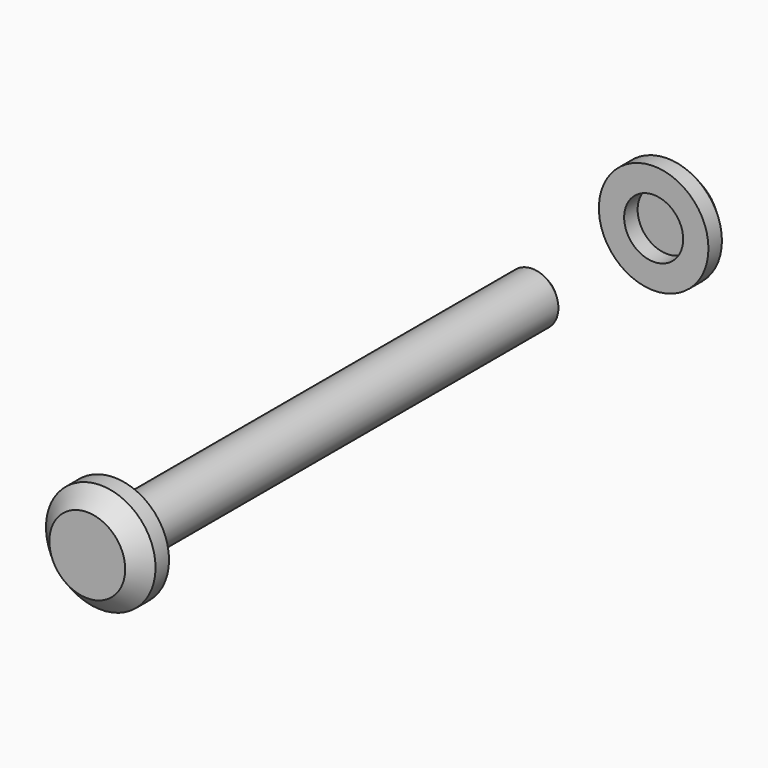
from build123d import *

# Parameters (mm, degrees)
F0_R     = 1.55
F1_DEPTH = 31.5
F0_R_2   = 3.25
F0_R_3   = 1.75
F2_DEPTH = 2
F3_SIZE  = 1
F4_SIZE  = 0.5
F5_START = -40
F5_DEPTH = 2
F6_START = -41
F6_DEPTH = 1
F7_SIZE  = 1


with BuildPart() as f1:
    # F0 (on Front) → F1 (new body)
    with BuildSketch(Plane.XZ):
        Circle(F0_R)
    extrude(amount=-F1_DEPTH)

    # F0 (on Front) → F2 (join)
    with BuildSketch(Plane.XZ):
        Circle(F0_R_2)
        Circle(F0_R_3, mode=Mode.SUBTRACT)
        Circle(F0_R_3)
        Circle(F0_R, mode=Mode.SUBTRACT)
        Circle(F0_R)
    extrude(amount=F2_DEPTH)

    # F3
    f3_edges = [f1.edges().sort_by_distance(p)[0] for p in [
        (-3.25, -2, 0),
    ]]
    chamfer(f3_edges, length=F3_SIZE)

    # F4
    f4_edges = [f1.edges().sort_by_distance(p)[0] for p in [
        (-1.55, 31.5, 0),
    ]]
    chamfer(f4_edges, length=F4_SIZE)


with BuildPart() as f5:
    # F0 (on Front) → F5 (new body)
    with BuildSketch(Plane.XZ.offset(F5_START)):
        Circle(F0_R_2)
        Circle(F0_R_3, mode=Mode.SUBTRACT)
    extrude(amount=-F5_DEPTH)

    # F0 (on Front) → F6 (join)
    with BuildSketch(Plane.XZ.offset(F6_START)):
        Circle(F0_R_3)
        Circle(F0_R, mode=Mode.SUBTRACT)
        Circle(F0_R)
    extrude(amount=-F6_DEPTH)

    # F7
    f7_edges = [f5.edges().sort_by_distance(p)[0] for p in [
        (-3.25, 42, 0),
    ]]
    chamfer(f7_edges, length=F7_SIZE)


solid = Compound([f1.part, f5.part])
